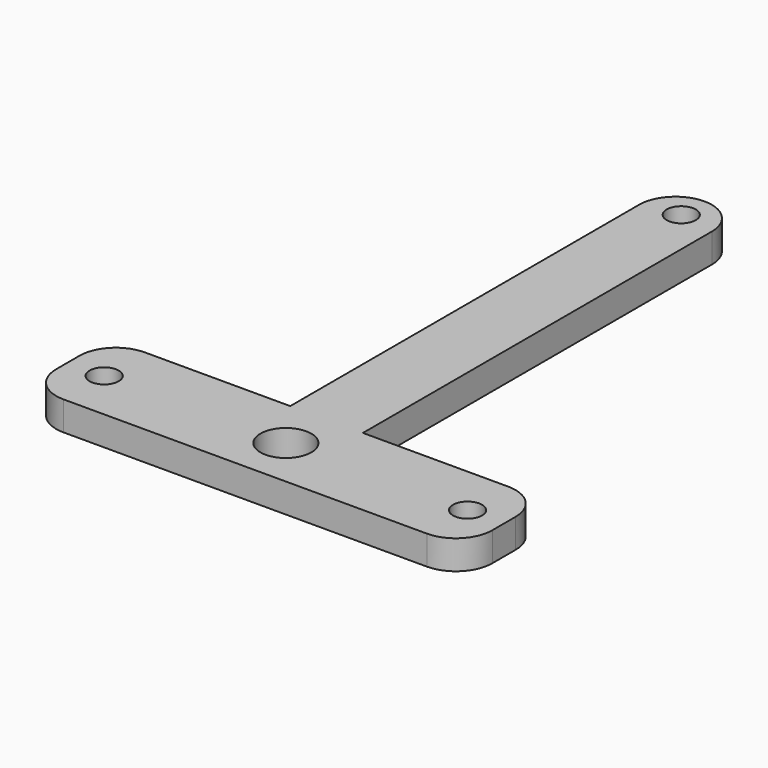
from build123d import *

# Parameters (mm, degrees)
F1_DEPTH = 4
F2_R     = 2
F2_R_2   = 3.5
F3_DEPTH = 25
F4_R     = 4.99999


# Not quite as in the source:
# - a fillet or chamfer is up to 0.001 mm smaller than in the source, because OpenCascade refuses the exact size


with BuildPart() as f1:
    # F0 (on Top) → F1 (new body)
    with BuildSketch(Plane.XY):
        Polygon((-5, 65), (-5, 0), (-30, 0), (-30, -14), (30, -14), (30, 0), (5, 0), (5, 65), align=None)
    extrude(amount=F1_DEPTH)

    # F2 (on face) → F3 (cut)
    with BuildSketch(Plane.XY.offset(4)):
        with Locations((-25, -7)):
            Circle(F2_R)
        with Locations((25, -7)):
            Circle(F2_R)
        with Locations((0, -7)):
            Circle(F2_R_2)
        with Locations((0, 61)):
            Circle(F2_R)
    extrude(amount=-F3_DEPTH, mode=Mode.SUBTRACT)

    # F4 (radius 5 in the source; OpenCascade refuses exactly that, so slightly less here)
    f4_edges = [f1.edges().sort_by_distance(p)[0] for p in [
        (-30, -14, 2),
        (-30, 0, 2),
        (30, -14, 2),
        (30, 0, 2),
        (5, 65, 2),
        (-5, 65, 2),
    ]]
    fillet(f4_edges, radius=F4_R)


solid = f1.part
